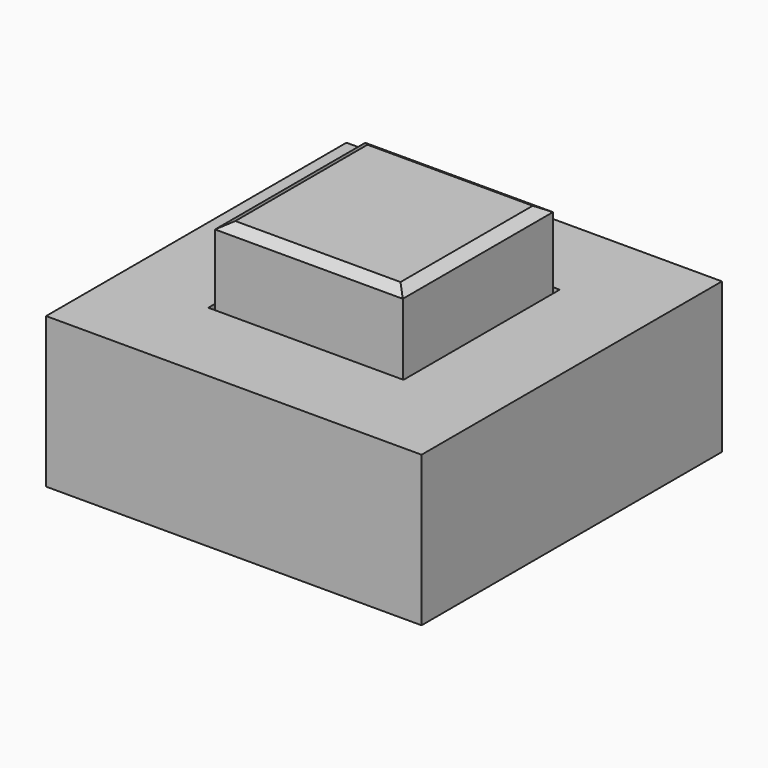
from build123d import *

# Parameters (mm, degrees)
F0_W        = 10
F0_H        = 10
F1_DEPTH    = 12
F0_W_2      = 20
F0_H_2      = 20
F0_W_3      = 10.4
F0_H_3      = 10.4
F2_DEPTH    = 8
F3_C1_SIZE2 = 0.6
F3_C1_SIZE  = 0.3464101615
F3_C2_SIZE2 = 0.6
F3_C2_SIZE  = 0.3464101615
F3_C3_SIZE2 = 0.3464101615
F3_C3_SIZE  = 0.6
F3_C4_SIZE2 = 0.6
F3_C4_SIZE  = 0.3464101615
F3_C5_SIZE2 = 0.6
F3_C5_SIZE  = 0.3464101615
F3_C6_SIZE2 = 0.6
F3_C6_SIZE  = 0.3464101615
F3_C7_SIZE2 = 0.6
F3_C7_SIZE  = 0.3464101615
F3_C8_SIZE2 = 0.6
F3_C8_SIZE  = 0.3464101615


with BuildPart() as f1:
    # F0 (on Top) → F1 (new body)
    with BuildSketch(Plane.XY):
        Rectangle(F0_W, F0_H)
    extrude(amount=F1_DEPTH)

    # F3: chamfer of 0.6 x 0.3464101615 on 8 edges, made by hand

    # F3_c1
    f3_c1_edges = [f1.edges().sort_by_distance(p)[0] for p in [
        (5, 0, 0),
    ]]
    f3_c1_side = f1.faces().sort_by_distance((5, 0, 0.0069282032))[0]
    chamfer(f3_c1_edges, length=F3_C1_SIZE, length2=F3_C1_SIZE2, reference=f3_c1_side)

    # F3_c2
    f3_c2_edges = [f1.edges().sort_by_distance(p)[0] for p in [
        (5, 0, 12),
    ]]
    f3_c2_side = f1.faces().sort_by_distance((5, 0, 11.9930717968))[0]
    chamfer(f3_c2_edges, length=F3_C2_SIZE, length2=F3_C2_SIZE2, reference=f3_c2_side)

    # F3_c3
    f3_c3_edges = [f1.edges().sort_by_distance(p)[0] for p in [
        (-0.3, 5, 0),
    ]]
    f3_c3_side = f1.faces().sort_by_distance((-0.3, 5, 0.0069282032))[0]
    chamfer(f3_c3_edges, length=F3_C3_SIZE, length2=F3_C3_SIZE2, reference=f3_c3_side)

    # F3_c4
    f3_c4_edges = [f1.edges().sort_by_distance(p)[0] for p in [
        (-0.3, 5, 12),
    ]]
    f3_c4_side = f1.faces().sort_by_distance((-0.3, 5, 11.9930717968))[0]
    chamfer(f3_c4_edges, length=F3_C4_SIZE, length2=F3_C4_SIZE2, reference=f3_c4_side)

    # F3_c5
    f3_c5_edges = [f1.edges().sort_by_distance(p)[0] for p in [
        (-5, -0.1732050808, 0),
    ]]
    f3_c5_side = f1.faces().sort_by_distance((-5, -0.1732050808, 0.0069282032))[0]
    chamfer(f3_c5_edges, length=F3_C5_SIZE, length2=F3_C5_SIZE2, reference=f3_c5_side)

    # F3_c6
    f3_c6_edges = [f1.edges().sort_by_distance(p)[0] for p in [
        (-5, -0.3, 12),
    ]]
    f3_c6_side = f1.faces().sort_by_distance((-5, -0.3, 11.9930717968))[0]
    chamfer(f3_c6_edges, length=F3_C6_SIZE, length2=F3_C6_SIZE2, reference=f3_c6_side)

    # F3_c7
    f3_c7_edges = [f1.edges().sort_by_distance(p)[0] for p in [
        (0, -5, 0),
    ]]
    f3_c7_side = f1.faces().sort_by_distance((0, -5, 0.0069282032))[0]
    chamfer(f3_c7_edges, length=F3_C7_SIZE, length2=F3_C7_SIZE2, reference=f3_c7_side)

    # F3_c8
    f3_c8_edges = [f1.edges().sort_by_distance(p)[0] for p in [
        (0, -5, 12),
    ]]
    f3_c8_side = f1.faces().sort_by_distance((0, -5, 11.9930717968))[0]
    chamfer(f3_c8_edges, length=F3_C8_SIZE, length2=F3_C8_SIZE2, reference=f3_c8_side)


with BuildPart() as f2:
    # F0 (on Top) → F2 (new body)
    with BuildSketch(Plane.XY):
        Rectangle(F0_W_2, F0_H_2)
        Rectangle(F0_W_3, F0_H_3, mode=Mode.SUBTRACT)
    extrude(amount=F2_DEPTH)


solid = Compound([f1.part, f2.part])
